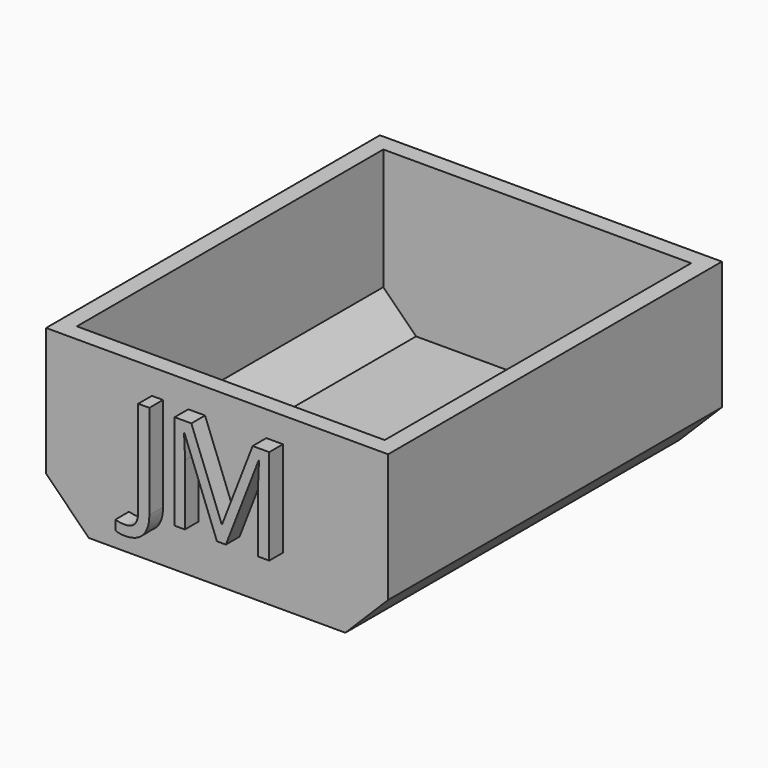
from build123d import *

# Parameters (mm, degrees)
F1_DEPTH     = 61.976
F2_T         = -2.54
F3_TEXT_SIZE = 19.8727201981
F4_DEPTH     = 2.54


# Not quite as in the source:
# - Text() gives the source's letters only with a copy of the font that has no kerning and outlines rounded to 1/6400 em; it was checked with that copy


with BuildPart() as f1:
    # F0 (on Front) → F1 (new body)
    with BuildSketch(Plane.XZ):
        Polygon((0, 6.35), (6.35, 0), (44.45, 0), (50.8, 6.35), (50.8, 25.4), (0, 25.4), align=None)
    extrude(amount=F1_DEPTH)

    # F2
    f2_openings = [f1.faces().sort_by_distance(p)[0] for p in [
        (25.4, -30.988, 25.4),
    ]]
    offset(amount=F2_T, openings=f2_openings)

    # F3 (on face) → F4 (join)
    with BuildSketch(Plane.XZ.offset(61.976)):
        with Locations((13.8703454286, 7.4461875483)):
            Text('JM', F3_TEXT_SIZE, font='Open Sans', text_align=(TextAlign.LEFT, TextAlign.BOTTOM))
    extrude(amount=F4_DEPTH)


solid = f1.part
